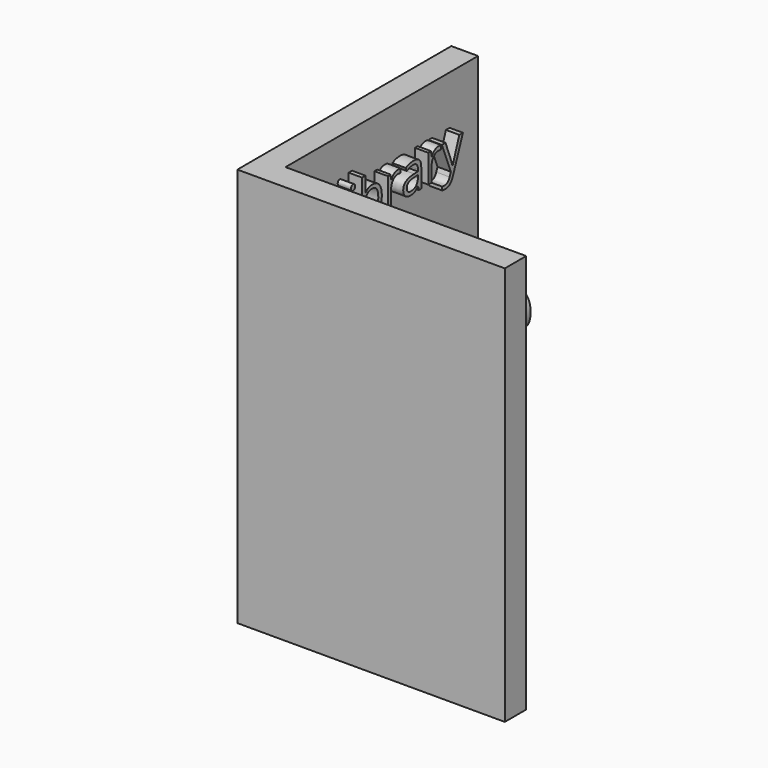
from build123d import *

# Parameters (mm, degrees)
F0_W         = 50.8
F0_H         = 75.8388625592
F1_DEPTH     = 5.08
F2_W         = 5.08
F2_H         = 75.8388625592
F3_DEPTH     = 45.72
F4_TEXT_SIZE = 9.9749485445
F6_DEPTH     = 2.54
F5_TEXT_SIZE = 9.9724287995
F7_DEPTH     = 2.54


# Not quite as in the source:
# - Text() gives the source's letters only with a copy of the font that has no kerning and outlines rounded to 1/6400 em; it was checked with that copy


with BuildPart() as f1:
    # F0 (on Right) → F1 (new body)
    with BuildSketch(Plane.YZ):
        Rectangle(F0_W, F0_H)
    extrude(amount=F1_DEPTH)

    # F2 (on face) → F3 (join)
    with BuildSketch(Plane.YZ.offset(5.08)):
        with Locations((-22.86, 0)):
            Rectangle(F2_W, F2_H)
    extrude(amount=F3_DEPTH)

    # F4 (on face) → F6 (join)
    with BuildSketch(Plane(origin=(0, -20.32, 0), x_dir=(-1, 0, 0), z_dir=(0, 1, 0))):
        with Locations((-50.2225570381, 23.5302392393)):
            Text('Oakmont', F4_TEXT_SIZE, font='Open Sans', text_align=(TextAlign.LEFT, TextAlign.BOTTOM))
    extrude(amount=F6_DEPTH)

    # F5 (on face) → F7 (join)
    with BuildSketch(Plane.YZ.offset(5.08)):
        with Locations((-13.8830659853, 23.3223382384)):
            Text('Library', F5_TEXT_SIZE, font='Open Sans', text_align=(TextAlign.LEFT, TextAlign.BOTTOM))
    extrude(amount=F7_DEPTH)


solid = f1.part
